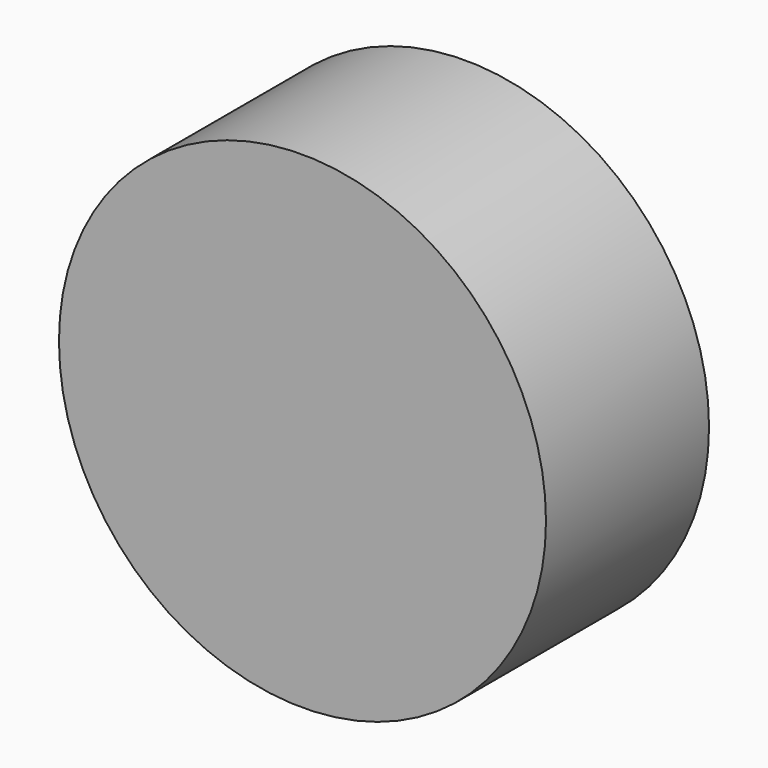
from build123d import *

# Parameters (mm, degrees)
F0_R     = 60.6949615143
F1_DEPTH = 50.8


# Not quite as in the source:
# - the program builds the solid bodies; features that only make, move or delete a surface that nothing else refers to are left out


with BuildPart() as f1:
    # F0 (on Front) → F1 (new body)
    with BuildSketch(Plane.XZ):
        Circle(F0_R)
    extrude(amount=F1_DEPTH)


solid = f1.part
